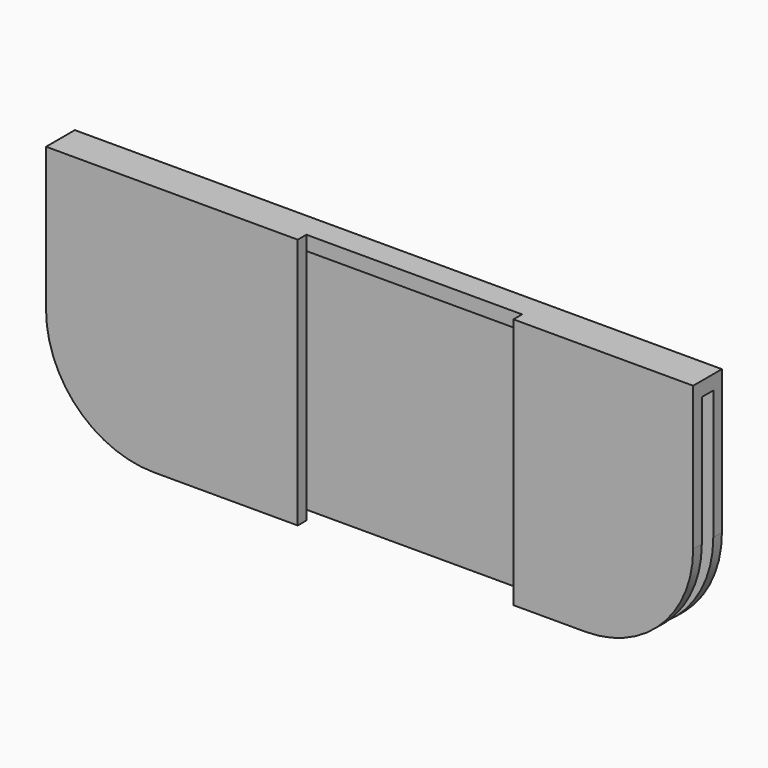
from build123d import *

# Parameters (mm, degrees)
F0_W     = 90
F0_H     = 35
F1_DEPTH = 5
F3_R     = 15
F2_W     = 2
F2_H     = 33
F4_DEPTH = 90
F5_W     = 30
F5_H     = 35
F6_DEPTH = 1.5


with BuildPart() as f1:
    # F0 (on Front) → F1 (new body)
    with BuildSketch(Plane.XZ):
        with Locations((-2.3338645697, 1.2048181861)):
            Rectangle(F0_W, F0_H)
    extrude(amount=F1_DEPTH)

    # F3
    f3_edges = [f1.edges().sort_by_distance(p)[0] for p in [
        (42.666135, -2.5, -16.295182),
        (-47.333865, -2.5, -16.295182),
    ]]
    fillet(f3_edges, radius=F3_R)

    # F2 (on face) → F4 (cut)
    with BuildSketch(Plane(origin=(-47.3338645697, 0, 0), x_dir=(0, -1, 0), z_dir=(-1, 0, 0))):
        with Locations((2.5, 0.2048181861)):
            Rectangle(F2_W, F2_H)
    extrude(amount=-F4_DEPTH, mode=Mode.SUBTRACT)

    # F5 (on face) → F6 (cut)
    with BuildSketch(Plane.XZ.offset(5)):
        with Locations((2.6661354303, 1.2048181861)):
            Rectangle(F5_W, F5_H)
    extrude(amount=-F6_DEPTH, mode=Mode.SUBTRACT)


solid = f1.part
